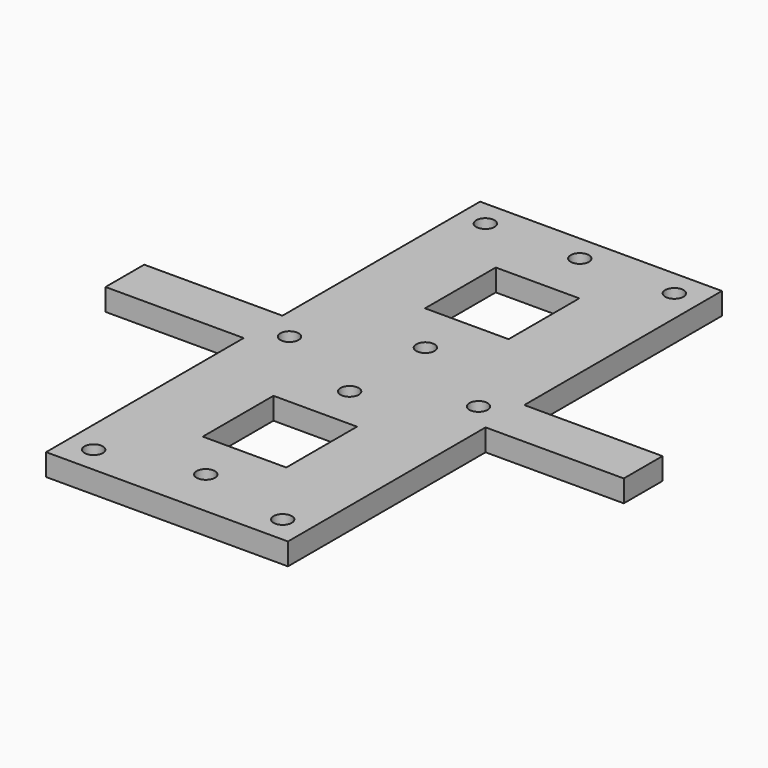
from build123d import *

# Parameters (mm, degrees)
F0_W      = 22.25
F0_H      = 17.875
F1_DEPTH  = 3.175
F2_DEPTH  = 5.08
F3_DEPTH  = 2.54
F4_DEPTH  = 5.08
F5_DEPTH  = 5.08
F6_DEPTH  = 5.08
F7_DEPTH  = 4.7498
F8_DEPTH  = 4.7498
F9_DEPTH  = 4.7498
F10_DEPTH = 4.7498
F11_DEPTH = 2.54
F12_R     = 1.325
F13_DEPTH = 25.4
F14_DEPTH = 25.4
F15_DEPTH = 25.4
F16_DEPTH = 25.4


# Not quite as in the source:
# - a feature names something its author has since deleted; it is built from what else it names


with BuildPart() as f1:
    # F0 (on Top) → F1 (new body)
    with BuildSketch(Plane.XY):
        Polygon((0, 35.75), (0, 0), (44.5, 0), (44.5, 35.75), (64.5, 35.75), (64.5, 39.25), (64.5, 42.75), (44.5, 42.75), (44.5, 78.5), (0, 78.5), (0, 42.75), (-20, 42.75), (-20, 39.25), (-20, 35.75), align=None)
        with Locations((22.25, 17.875)):
            Rectangle(F0_W, F0_H, mode=Mode.SUBTRACT)
        with Locations((22.25, 60.625)):
            Rectangle(F0_W, F0_H, mode=Mode.SUBTRACT)
    extrude(amount=F1_DEPTH)

    # F2 (add): a face of the model
    f2_faces = [f1.faces().sort_by_distance(p)[0] for p in [
        (22.25, 69.5625, 1.5875),
    ]]
    extrude(f2_faces, amount=F2_DEPTH)

    # F3 (add): faces of the model
    f3_faces = [f1.faces().sort_by_distance(p)[0] for p in [
        (22.25, 51.6875, 1.5875),
        (22.25, 26.8125, 1.5875),
    ]]
    extrude(f3_faces, amount=F3_DEPTH, dir=(0, 1, 0))

    # F4 (add): a face of the model
    f4_faces = [f1.faces().sort_by_distance(p)[0] for p in [
        (22.25, 8.9375, 1.5875),
    ]]
    extrude(f4_faces, amount=F4_DEPTH)

    # F5 (add): faces of the model
    f5_faces = [f1.faces().sort_by_distance(p)[0] for p in [
        (33.375, 59.355, 1.5875),
        (33.375, 20.415, 1.5875),
    ]]
    extrude(f5_faces, amount=F5_DEPTH)

    # F6 (add): faces of the model
    f6_faces = [f1.faces().sort_by_distance(p)[0] for p in [
        (11.125, 59.355, 1.5875),
        (11.125, 20.415, 1.5875),
    ]]
    extrude(f6_faces, amount=F6_DEPTH)

    # F7 (cut): faces of the model
    f7_faces = [f1.faces().sort_by_distance(p)[0] for p in [
        (44.5, 60.625, 1.5875),
        (44.5, 17.875, 1.5875),
    ]]
    extrude(f7_faces, amount=-F7_DEPTH, mode=Mode.SUBTRACT)

    # F8 (cut): faces of the model
    f8_faces = [f1.faces().sort_by_distance(p)[0] for p in [
        (0, 60.625, 1.5875),
        (0, 17.875, 1.5875),
    ]]
    extrude(f8_faces, amount=-F8_DEPTH, mode=Mode.SUBTRACT)

    # F9 (cut): a face of the model
    f9_faces = [f1.faces().sort_by_distance(p)[0] for p in [
        (-20, 39.25, 1.5875),
    ]]
    extrude(f9_faces, amount=-F9_DEPTH, mode=Mode.SUBTRACT)

    # F10 (cut): a face of the model
    f10_faces = [f1.faces().sort_by_distance(p)[0] for p in [
        (64.5, 39.25, 1.5875),
    ]]
    extrude(f10_faces, amount=-F10_DEPTH, mode=Mode.SUBTRACT)

    # F11 (cut): a face of the model
    f11_faces = [f1.faces().sort_by_distance(p)[0] for p in [
        (22.25, 64.4825, 1.5875),
    ]]
    extrude(f11_faces, amount=-F11_DEPTH, mode=Mode.SUBTRACT)

    # F12 (on face) → F13 (cut)
    with BuildSketch(Plane(origin=(0, 0, 0), x_dir=(1, 0, 0), z_dir=(0, 0, -1))):
        with BuildLine():
            ThreePointArc((34.6002, -74.675), (35.9252, -76), (37.2502, -74.675))
            ThreePointArc((37.2502, -74.675), (35.9252, -73.35), (34.6002, -74.675))
        make_face()
        with Locations((8.5748, -74.675)):
            Circle(F12_R)
        with Locations((8.5748, -39.25)):
            Circle(F12_R)
        with BuildLine():
            ThreePointArc((34.6002, -39.25), (35.9252, -40.575), (37.2502, -39.25))
            ThreePointArc((37.2502, -39.25), (35.9252, -37.925), (34.6002, -39.25))
        make_face()
        with Locations((35.9252, -3.825)):
            Circle(F12_R)
        with Locations((8.5748, -3.825)):
            Circle(F12_R)
    extrude(amount=-F13_DEPTH, mode=Mode.SUBTRACT)

    # F12 (on face) → F14 (cut)
    with BuildSketch(Plane(origin=(0, 0, 0), x_dir=(1, 0, 0), z_dir=(0, 0, -1))):
        with Locations((22.25, -74.675)):
            Circle(F12_R)
    extrude(amount=-F14_DEPTH, mode=Mode.SUBTRACT)

    # F12 (on face) → F15 (cut)
    with BuildSketch(Plane(origin=(0, 0, 0), x_dir=(1, 0, 0), z_dir=(0, 0, -1))):
        with Locations((22.25, -7.00875)):
            Circle(F12_R)
        with Locations((22.25, -46.73875)):
            Circle(F12_R)
    extrude(amount=-F15_DEPTH, mode=Mode.SUBTRACT)

    # F12 (on face) → F16 (cut)
    with BuildSketch(Plane(origin=(0, 0, 0), x_dir=(1, 0, 0), z_dir=(0, 0, -1))):
        with Locations((22.25, -33.03125)):
            Circle(F12_R)
    extrude(amount=-F16_DEPTH, mode=Mode.SUBTRACT)


solid = f1.part
